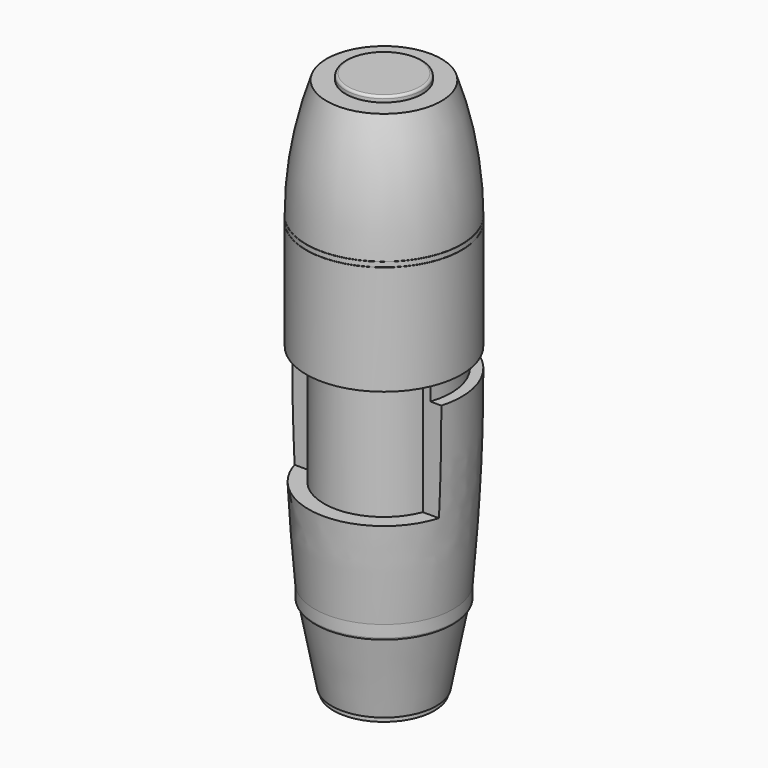
from build123d import *

# Parameters (mm, degrees)
F3_DEPTH = 25
F4_R     = 0.5
F7_R     = 0.49999


# Not quite as in the source:
# - a fillet or chamfer is up to 0.001 mm smaller than in the source, because OpenCascade refuses the exact size


with BuildPart() as f1:
    # F0 (on Front) → F1 (revolve)
    with BuildSketch(Plane.XZ):
        with BuildLine():
            Line((-14.5, 0), (0, 0))
            Line((0, 0), (0, 94))
            Line((0, 94), (-8, 94))
            Line((-8, 94), (-8, 92.8))
            Line((-8, 92.8), (-12, 92.8))
            ThreePointArc((-12, 92.8), (-15.1799323999, 80.479338508), (-16.25, 67.8))
            Line((-16.25, 67.8), (-16.05, 67.8))
            Line((-16.05, 67.8), (-16.05, 67.75))
            Line((-16.05, 67.75), (-16.25, 67.75))
            Line((-16.25, 67.75), (-16.25, 66.75))
            Line((-16.25, 66.75), (-16.05, 66.75))
            Line((-16.05, 66.75), (-16.05, 66.7))
            Line((-16.05, 66.7), (-16.25, 66.7))
            Line((-16.25, 66.7), (-16.25, 43.8))
            Line((-16.25, 43.8), (-14.05, 43.8))
            Line((-14.05, 43.8), (-14.05, 39.7))
            Line((-14.05, 39.7), (-16.25, 39.7))
            ThreePointArc((-16.25, 39.7), (-15.8122876797, 19.8307240947), (-14.5, 0))
        make_face()
    revolve(axis=Axis((0, 0, 47), (0, 0, 1)))

    # F2 (on face) → F3 (cut)
    with BuildSketch(Plane(origin=(0, 0, 43.8), x_dir=(1, 0, 0), z_dir=(0, 0, -1))):
        with BuildLine():
            Line((11.7154812108, 4.5), (15.6144964696, 4.5))
            ThreePointArc((15.6144964696, 4.5), (0, 16.25), (-15.6144964696, 4.5))
            Line((-15.6144964696, 4.5), (-11.7154812108, 4.5))
            ThreePointArc((-11.7154812108, 4.5), (0, 12.55), (11.7154812108, 4.5))
        make_face()
    extrude(amount=F3_DEPTH, mode=Mode.SUBTRACT)

    # F4
    f4_edges = [f1.edges().sort_by_distance(p)[0] for p in [
        (8, 0, 94),
    ]]
    fillet(f4_edges, radius=F4_R)

    # F5 (on Front) → F6 (revolve)
    with BuildSketch(Plane.XZ):
        Polygon((14.5, 0), (0, 0), (0, -20), (10.55, -20), (10.55, -19), (10.95, -19), (14, -3), (14.5, -3), align=None)
    revolve(axis=Axis((0, 0, -10), (0, 0, -1)))

    # F7 (radius 0.5 in the source; OpenCascade refuses exactly that, so slightly less here)
    f7_edges = [f1.edges().sort_by_distance(p)[0] for p in [
        (-14.5, 0, -3),
    ]]
    fillet(f7_edges, radius=F7_R)


solid = f1.part
